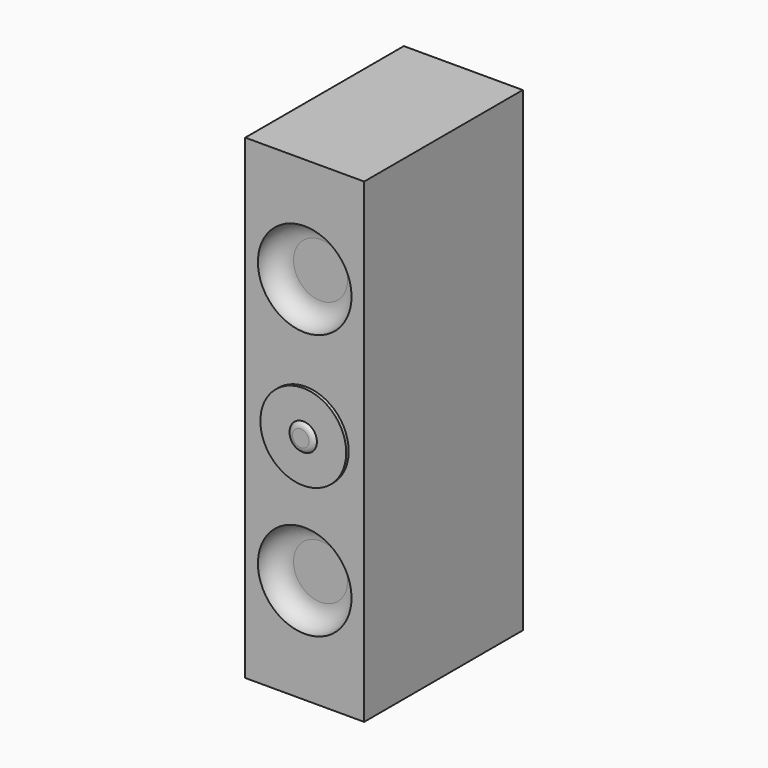
from build123d import *

# Parameters (mm, degrees)
F0_W     = 152.4
F0_H     = 254
F1_DEPTH = 609.6
F3_DEPTH = 25.4
F4_R     = 25.39999
F5_DEPTH = 4
F6_DEPTH = 8


# Not quite as in the source:
# - a fillet or chamfer that OpenCascade refuses, or shapes differently, is made with other operations: its cross-section is extruded or revolved along the edge and cut away or added
# - a fillet or chamfer is up to 0.001 mm smaller than in the source, because OpenCascade refuses the exact size


with BuildPart() as f1:
    # F0 (on Top) → F1 (new body)
    with BuildSketch(Plane.XY):
        with Locations((76.2, 127)):
            Rectangle(F0_W, F0_H)
    extrude(amount=F1_DEPTH)

    # F2 (on face) → F3 (cut)
    with BuildSketch(Plane.XZ):
        with BuildLine():
            Line((76.2, 414.5332613452), (76.2, 534.5332613452))
            ThreePointArc((76.2, 534.5332613452), (16.2, 474.5332613452), (76.2, 414.5332613452))
        make_face()
        with BuildLine():
            ThreePointArc((76.2, 414.5332613452), (118.6264068712, 432.106854474), (136.2, 474.5332613452))
            ThreePointArc((136.2, 474.5332613452), (118.6264068712, 516.9596682164), (76.2, 534.5332613452))
            Line((76.2, 534.5332613452), (76.2, 414.5332613452))
        make_face()
        with BuildLine():
            Line((76.2, 74.5332613452), (76.2, 194.5332613452))
            ThreePointArc((76.2, 194.5332613452), (16.2, 134.5332613452), (76.2, 74.5332613452))
        make_face()
        with BuildLine():
            ThreePointArc((136.2, 134.5332613452), (118.6264068712, 176.9596682164), (76.2, 194.5332613452))
            Line((76.2, 194.5332613452), (76.2, 74.5332613452))
            ThreePointArc((76.2, 74.5332613452), (118.6264068712, 92.106854474), (136.2, 134.5332613452))
        make_face()
    extrude(amount=-F3_DEPTH, mode=Mode.SUBTRACT)

    # F4 (radius 25.4 in the source; OpenCascade refuses exactly that, so slightly less here)
    f4_edges = [f1.edges().sort_by_distance(p)[0] for p in [
        (76.2, 25.4, 534.533261),
        (76.2, 25.4, 194.533261),
    ]]
    fillet(f4_edges, radius=F4_R)

    # F2 (on face) → F5 (join)
    with BuildSketch(Plane.XZ):
        with BuildLine():
            ThreePointArc((132.5678679347, 298.8973259926), (115.9720816592, 338.2688432126), (76.2, 353.8803137007))
            Line((76.2, 353.8803137007), (76.2, 316.3437851552))
            ThreePointArc((76.2, 316.3437851552), (89.4487835379, 311.7462109414), (95.0678679347, 298.8973259926))
            ThreePointArc((95.0678679347, 298.8973259926), (89.4487835379, 286.0484410437), (76.2, 281.45086683))
            Line((76.2, 281.45086683), (76.2, 243.9143382844))
            ThreePointArc((76.2, 243.9143382844), (115.9720816592, 259.5258087726), (132.5678679347, 298.8973259926))
        make_face()
        with BuildLine():
            Line((76.2, 316.3437851552), (76.2, 353.8803137007))
            ThreePointArc((76.2, 353.8803137007), (22.5678679347, 298.8973259926), (76.2, 243.9143382844))
            Line((76.2, 243.9143382844), (76.2, 281.45086683))
            ThreePointArc((76.2, 281.45086683), (60.0678679347, 298.8973259926), (76.2, 316.3437851552))
        make_face()
    extrude(amount=F5_DEPTH)

    # F2 (on face) → F6 (join)
    with BuildSketch(Plane.XZ):
        with BuildLine():
            ThreePointArc((95.0678679347, 298.8973259926), (89.4487835379, 311.7462109414), (76.2, 316.3437851552))
            Line((76.2, 316.3437851552), (76.2, 281.45086683))
            ThreePointArc((76.2, 281.45086683), (89.4487835379, 286.0484410437), (95.0678679347, 298.8973259926))
        make_face()
        with BuildLine():
            Line((76.2, 281.45086683), (76.2, 316.3437851552))
            ThreePointArc((76.2, 316.3437851552), (60.0678679347, 298.8973259926), (76.2, 281.45086683))
        make_face()
    extrude(amount=F6_DEPTH)

    # F7: fillet of radius 8 on 1 edges, made by hand

    # F7_s1 → F7_t2 (revolve, cut)
    with BuildSketch(Plane.XY.offset(298.8973259926)):
        with BuildLine():
            ThreePointArc((95.0678679347, -4), (92.1396647044, -6.9282032303), (88.1396647044, -8))
            Line((88.1396647044, -8), (95.0678679347, -8))
            Line((95.0678679347, -8), (95.0678679347, -4))
        make_face()
    revolve(axis=Axis((77.5678679347, -8, 298.8973259926), (0, -1, 0)), mode=Mode.SUBTRACT)


solid = f1.part
